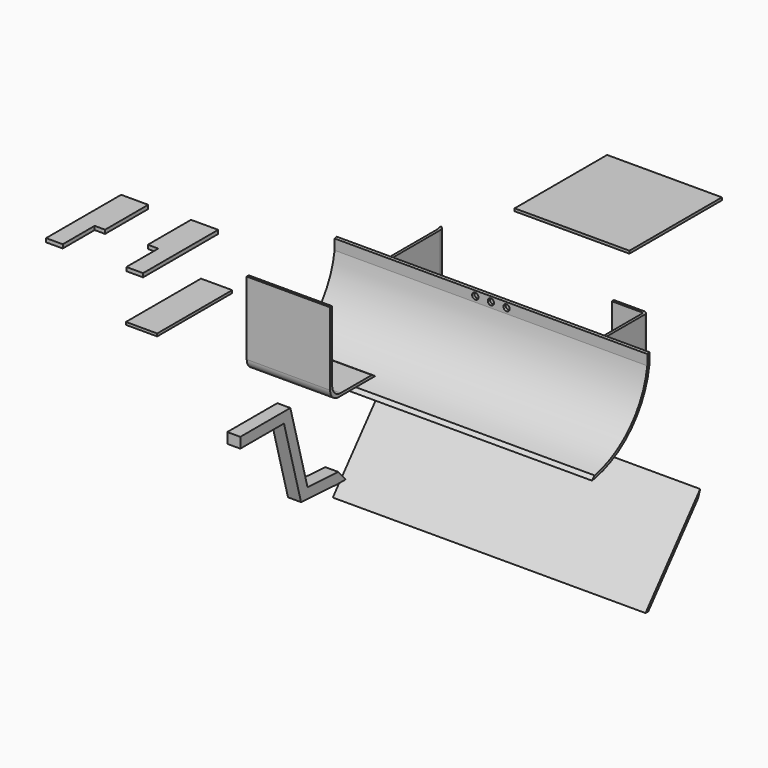
from build123d import *

# Parameters (mm, degrees)
F1_DEPTH  = 190.5
F2_W      = 19.05
F2_H      = 57.15
F3_DEPTH  = 1.6002
F5_DEPTH  = 190.5
F7_DEPTH  = 50.8
F8_W      = 69.9347853661
F8_H      = 70.4333484173
F21_DEPTH = 1.6002
F22_DEPTH = 7.9375
F10_R     = 1.905
F11_DEPTH = 83.3087024486
F13_DEPTH = 2.286
F15_DEPTH = 2.286
F16_W     = 1.6002
F16_H     = 31.75
F19_W     = 9.6304351464
F19_H     = 31.75
F20_DEPTH = 25.4


# Not quite as in the source:
# - a feature names something its author has since deleted; it is built from what else it names


with BuildPart() as f1:
    # F0 (on Right) → F1 (new body)
    with BuildSketch(Plane.YZ):
        with BuildLine():
            Line((2.9455358163, 50.5775293171), (1.3453358163, 50.2454929949))
            Line((1.3453358163, 50.2454929949), (1.3453358163, 43.8954929949))
            ThreePointArc((1.3453358163, 43.8954929949), (-11.8950260011, 16.2331476976), (-38.7503645073, 1.4242543521))
            Line((-38.7503645073, 1.4242543521), (-40.7147916438, -0.59183615))
            Line((-40.7147916438, -0.59183615), (-38.4423047946, -0.1460129033))
            ThreePointArc((-38.4423047946, -0.1460129033), (-10.6937083452, 15.1746548691), (2.9455358163, 43.7872130318))
            Line((2.9455358163, 43.7872130318), (2.9455358163, 50.5775293171))
        make_face()
    extrude(amount=F1_DEPTH)

    # F10 (on face) → F11 (cut, through all)
    with BuildSketch(Plane(origin=(0, 2.9455358163, 0), x_dir=(-1, 0, 0), z_dir=(0, 1, 0))):
        with Locations((-95.25, 47.1823711745)):
            Circle(F10_R)
        with Locations((-85.725, 47.1823711745)):
            Circle(F10_R)
        with Locations((-104.775, 47.1823711745)):
            Circle(F10_R)
    extrude(amount=-F11_DEPTH, mode=Mode.SUBTRACT)


with BuildPart() as f3:
    # F2 (on Top) → F3 (new body)
    with BuildSketch(Plane.XY):
        with Locations((-72.6671729922, -26.2355463386)):
            Rectangle(F2_W, F2_H)
    extrude(amount=F3_DEPTH)


with BuildPart() as f5:
    # F4 (on Right) → F5 (new body)
    with BuildSketch(Plane.YZ):
        Polygon((40.0331534794, -42.9351368162), (41.6333534794, -38.5386234495), (0, -88.1553220304), (2.0889127444, -88.1553220304), align=None)
    extrude(amount=F5_DEPTH)


with BuildPart() as f7:
    # F6 (on Right) → F7 (new body)
    with BuildSketch(Plane.YZ):
        with BuildLine():
            Line((-63.957339463, 57.0222916961), (-65.557539463, 57.0222916961))
            Line((-65.557539463, 57.0222916961), (-65.557539463, 12.5722916961))
            ThreePointArc((-65.557539463, 12.5722916961), (-63.6976675236, 8.0821636355), (-59.207539463, 6.2222916961))
            Line((-59.207539463, 6.2222916961), (-33.807539463, 6.2222916961))
            Line((-33.807539463, 6.2222916961), (-31.1940032989, 6.2222916961))
            Line((-31.1940032989, 6.2222916961), (-33.807539463, 7.8224916961))
            Line((-33.807539463, 7.8224916961), (-57.607339463, 7.8224916961))
            ThreePointArc((-57.607339463, 7.8224916961), (-62.0974675236, 9.6823636355), (-63.957339463, 14.1724916961))
            Line((-63.957339463, 14.1724916961), (-63.957339463, 57.0222916961))
        make_face()
    extrude(amount=F7_DEPTH)


with BuildPart() as f21:
    # F8 (on Top) → F21 (new body)
    with BuildSketch(Plane.XY):
        with Locations((24.062409997, 187.307536602)):
            Rectangle(F8_W, F8_H)
    extrude(amount=F21_DEPTH)


with BuildPart() as f22:
    # F9 (on Right) → F22 (new body)
    with BuildSketch(Plane.YZ):
        Polygon((-42.2621666323, -20.3390651836), (-80.3621666323, -20.3390651836), (-80.3621666323, -26.6890651836), (-47.1078351951, -26.6890651836), (-34.1087002788, -74.1873922208), (-6.1264390171, -75.8113767203), (0, -75.8113767203), (-5.7585281372, -69.4720438228), (-29.1877967625, -68.1122977778), align=None)
    extrude(amount=F22_DEPTH)


with BuildPart() as f13:
    # F12 (on Top) → F13 (new body)
    with BuildSketch(Plane.XY):
        Polygon((-164.9733781815, 45.0218769178), (-164.9733781815, -12.1281230822), (-154.8133781815, -12.1281230822), (-154.8133781815, 12.1535500512), (-148.4633781815, 12.1535500512), (-148.4633781815, 45.0218769178), align=None)
    extrude(amount=F13_DEPTH)


with BuildPart() as f15:
    # F14 (on Top) → F15 (new body)
    with BuildSketch(Plane.XY):
        Polygon((-106.3901432657, -11.4971105634), (-106.3901432657, 45.6528894366), (-122.9001432657, 45.6528894366), (-122.9001432657, 12.7852894366), (-116.5501432657, 12.7852894366), (-116.5501432657, -11.4971105634), align=None)
    extrude(amount=F15_DEPTH)


with BuildPart() as f18:
    # F18: sweep along a path in F17
    with BuildLine(Plane.XY) as f18_path:
        Line((0, 69.313518703), (7.9582965779, 69.313518703))
        ThreePointArc((7.9582965779, 69.313518703), (9.5747426797, 68.6439648048), (10.2442965779, 67.027518703))
        Line((10.2442965779, 67.027518703), (10.2442965779, 29.689518703))
        ThreePointArc((10.2442965779, 29.689518703), (10.9138504761, 28.0730726012), (12.5302965779, 27.403518703))
        Line((12.5302965779, 27.403518703), (139.5302965779, 27.403518703))
        ThreePointArc((139.5302965779, 27.403518703), (141.1467426797, 28.0730726012), (141.8162965779, 29.689518703))
        Line((141.8162965779, 29.689518703), (141.8162965779, 60.169518703))
        ThreePointArc((141.8162965779, 60.169518703), (141.1467426797, 61.7859648048), (139.5302965779, 62.455518703))
        Line((139.5302965779, 62.455518703), (121.1970292659, 62.455518703))
    # F16 (on Right) → F18 (sweep)
    with BuildSketch(Plane.YZ):
        with Locations((69.9808419062, 15.875)):
            Rectangle(F16_W, F16_H)
    sweep(path=f18_path.line)

    # F19 (on face) → F20 (cut)
    with BuildSketch(Plane(origin=(0, 70.7809419062, 0), x_dir=(-1, 0, 0), z_dir=(0, 1, 0))):
        with Locations((-4.8152175732, 15.875)):
            Rectangle(F19_W, F19_H)
    extrude(amount=-F20_DEPTH, mode=Mode.SUBTRACT)


solid = Compound([f1.part, f3.part, f5.part, f7.part, f21.part, f22.part, f13.part, f15.part, f18.part])
